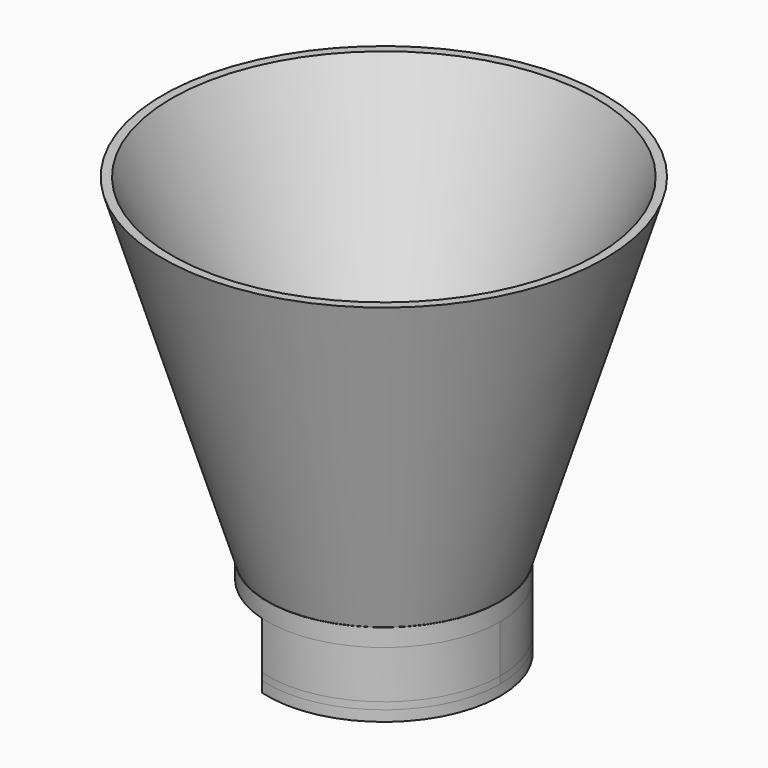
from build123d import *

# Parameters (mm, degrees)
F2_DEPTH      = 2
F3_R          = 12.15
F3_R_2        = 6.55
F4_DEPTH      = 2
F3_R_3        = 13.15
F5_DEPTH      = 6.2
F5_DEPTH_BACK = 2
F6_DEPTH      = 5.4
F6_DEPTH_BACK = 25
F7_SIZE       = 1
F8_T2_ANGLE   = 263.0691041821
F8_T4_ANGLE   = 263.0691041821
F11_R         = 13.1
F10_R         = 25
F13_R         = 24
F14_R         = 6.55


# Not quite as in the source:
# - a fillet or chamfer that OpenCascade refuses, or shapes differently, is made with other operations: its cross-section is extruded or revolved along the edge and cut away or added


with BuildPart() as f2:
    # F0 (on Top) → F2 (new body)
    with BuildSketch(Plane.XY):
        with BuildLine():
            ThreePointArc((-3.6462889984, -7.8439197178), (-8.65, 0), (-3.6462889984, 7.8439197178))
            Line((-3.6462889984, 7.8439197178), (-3.6462889984, 12.634360947))
            ThreePointArc((-3.6462889984, 12.634360947), (-13.15, 0), (-3.6462889984, -12.634360947))
            Line((-3.6462889984, -12.634360947), (-3.6462889984, -7.8439197178))
        make_face()
        with BuildLine():
            ThreePointArc((-3.6462889984, 7.8439197178), (4.6519942048, 7.2925612728), (8.65, 0))
            ThreePointArc((8.65, 0), (4.6519942048, -7.2925612728), (-3.6462889984, -7.8439197178))
            Line((-3.6462889984, -7.8439197178), (-3.6462889984, -12.634360947))
            ThreePointArc((-3.6462889984, -12.634360947), (7.9048655798, -10.5088343866), (13.15, 0))
            ThreePointArc((13.15, 0), (7.9048655798, 10.5088343866), (-3.6462889984, 12.634360947))
            Line((-3.6462889984, 12.634360947), (-3.6462889984, 7.8439197178))
        make_face()
    extrude(amount=-F2_DEPTH)



with BuildPart() as f4:
    # F3 (on offset) → F4 (new body)
    with BuildSketch(Plane.XY.offset(5.4)):
        Circle(F3_R)
        Circle(F3_R_2, mode=Mode.SUBTRACT)
    extrude(amount=F4_DEPTH)


with BuildPart() as f2_1:
    add(f2.part)

    add(f4.part)  # F5 merges F4
    # F3 (on offset) → F5 (join, two sides)
    with BuildSketch(Plane.XY.offset(5.4)) as f5_sk:
        Circle(F3_R_3)
        Circle(F3_R, mode=Mode.SUBTRACT)
    extrude(amount=-F5_DEPTH)
    extrude(f5_sk.sketch, amount=F5_DEPTH_BACK)

    # F0 (on Top) → F6 (cut, two sides)
    with BuildSketch(Plane.XY) as f6_sk:
        with BuildLine():
            ThreePointArc((-3.6462889984, -7.8439197178), (-8.65, 0), (-3.6462889984, 7.8439197178))
            Line((-3.6462889984, 7.8439197178), (-3.6462889984, 12.634360947))
            ThreePointArc((-3.6462889984, 12.634360947), (-13.15, 0), (-3.6462889984, -12.634360947))
            Line((-3.6462889984, -12.634360947), (-3.6462889984, -7.8439197178))
        make_face()
    extrude(amount=F6_DEPTH, mode=Mode.SUBTRACT)
    extrude(f6_sk.sketch, amount=-F6_DEPTH_BACK, mode=Mode.SUBTRACT)

    # F7
    f7_edges = [f2_1.edges().sort_by_distance(p)[0] for p in [
        (12.15, 0, 0),
    ]]
    chamfer(f7_edges, length=F7_SIZE)

    # F8: fillet of radius 1 on 2 edges, made by hand

    # F8_s1 → F8_t2 (revolve, cut)
    with BuildSketch(Plane(origin=(0, 0, 0), x_dir=(0, 0, 1), z_dir=(-0.7485559931, -0.6630715838, 0))):
        with BuildLine():
            ThreePointArc((0, 9.65), (-0.2928932188, 8.9428932188), (-1, 8.65))
            Line((-1, 8.65), (0, 8.65))
            Line((0, 8.65), (0, 9.65))
        make_face()
    revolve(axis=Axis((0, 0, 0), (0, 0, -1)), revolution_arc=F8_T2_ANGLE, mode=Mode.SUBTRACT)

    # F8_s3 → F8_t4 (revolve, cut)
    with BuildSketch(Plane(origin=(0, 0, 0), x_dir=(0, 0, 1), z_dir=(-0.7485559931, -0.6630715838, 0))):
        with BuildLine():
            ThreePointArc((-1, 8.65), (-1.7071067812, 8.9428932188), (-2, 9.65))
            Line((-2, 9.65), (-2, 8.65))
            Line((-2, 8.65), (-1, 8.65))
        make_face()
    revolve(axis=Axis((0, 0, -2), (0, 0, -1)), revolution_arc=F8_T4_ANGLE, mode=Mode.SUBTRACT)


with BuildPart() as f12:
    # F11 (on face) → F12 section 0
    with BuildSketch(Plane.XY.offset(7.4)):
        Circle(F11_R)
    # F10 (on offset) → F12 section 1
    with BuildSketch(Plane.XY.offset(45.4)):
        Circle(F10_R)
    loft()

    # F13 (on face) → F15 section 0
    with BuildSketch(Plane.XY.offset(45.4)):
        Circle(F13_R)
    # F14 (on face) → F15 section 1
    with BuildSketch(Plane.XY.offset(7.4)):
        Circle(F14_R)
    loft(mode=Mode.SUBTRACT)


solid = Compound([f2_1.part, f12.part])
